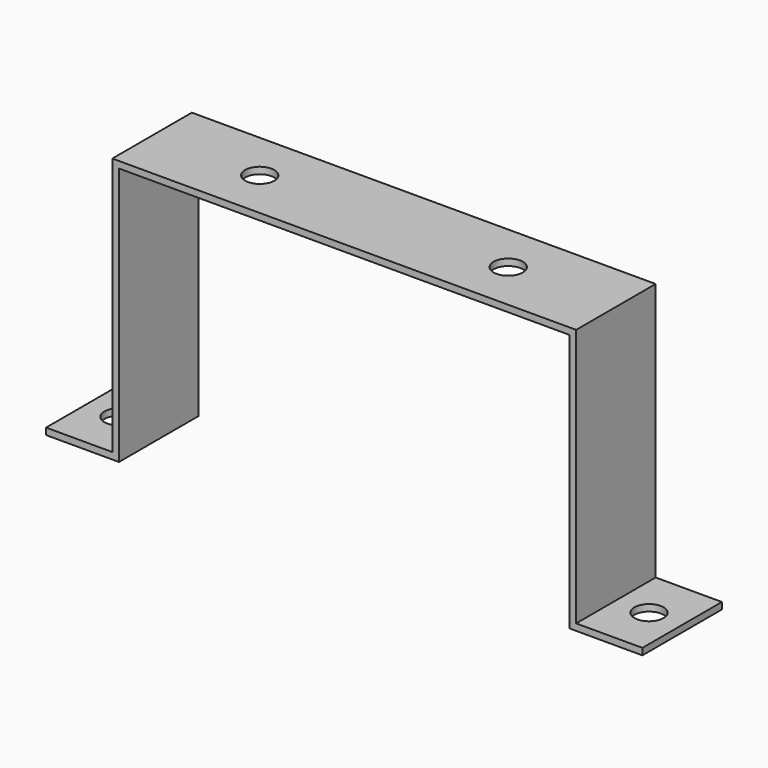
from build123d import *

# Parameters (mm, degrees)
F1_DEPTH = 30
F2_R     = 4.4
F3_R     = 4.4
F4_DEPTH = 25


# Not quite as in the source:
# - a feature names something its author has since deleted; it is built from what else it names


with BuildPart() as f1:
    # F0 (on Front) → F1 (new body)
    with BuildSketch(Plane.XZ):
        Polygon((90, -1), (90, 1), (70, 1), (70, 79), (-70, 79), (-70, 1), (-90, 1), (-90, -1), (-68, -1), (-68, 77), (68, 77), (68, -1), align=None)
    extrude(amount=F1_DEPTH)

    # F2 (on face) + F3 (on face) → F4 (cut)
    with BuildSketch(Plane.XY.offset(1)):
        with Locations((-80, -15)):
            Circle(F2_R)
        with Locations((80, -15)):
            Circle(F2_R)
    with BuildSketch(Plane.XY.offset(79)):
        with Locations((-37.5, -15)):
            Circle(F3_R)
        with Locations((37.5, -15)):
            Circle(F3_R)
    extrude(amount=-F4_DEPTH, mode=Mode.SUBTRACT)


solid = f1.part
